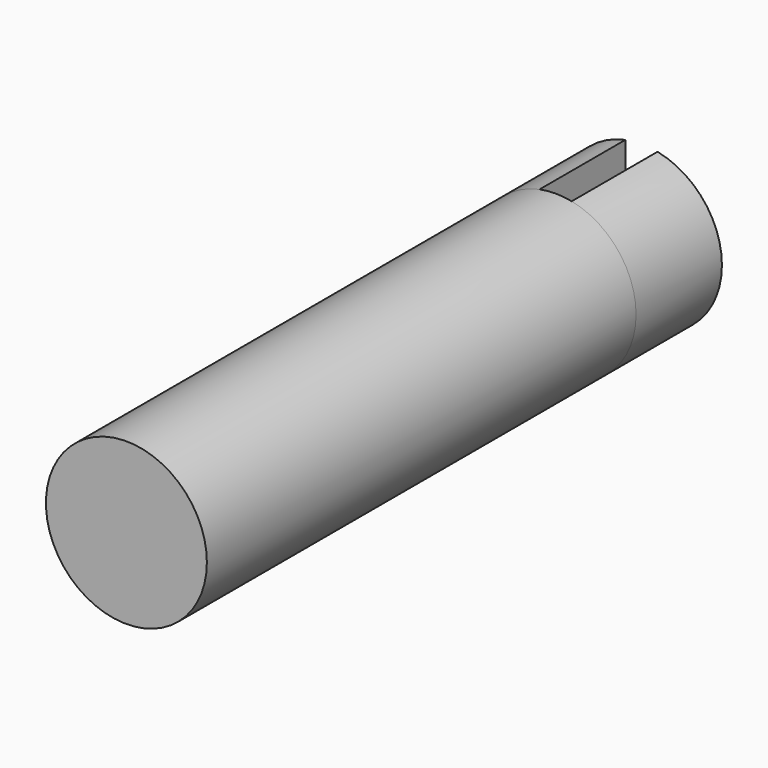
from build123d import *

# Parameters (mm, degrees)
F0_R     = 19.05
F1_DEPTH = 127
F3_DEPTH = 25.4


# Not quite as in the source:
# - after a boolean that leaves OpenCascade's solid faulty, fix() repairs it


with BuildPart() as f1:
    # F0 (on Front) → F1 (new body)
    with BuildSketch(Plane.XZ):
        Circle(F0_R)
    extrude(amount=F1_DEPTH)

    # F2 (on face) → F3 (join)
    with BuildSketch(Plane(origin=(0, 0, 0), x_dir=(-1, 0, 0), z_dir=(0, 1, 0))):
        with BuildLine():
            Line((-3.81, 11.045112), (-3.81, 18.665112))
            ThreePointArc((-3.81, 18.665112), (-19.05, 0), (-3.81, -18.665112))
            Line((-3.81, -18.665112), (-3.81, -11.045112))
            Line((-3.81, -11.045112), (3.81, -11.045112))
            Line((3.81, -11.045112), (3.81, -18.665112))
            ThreePointArc((3.81, -18.665112), (14.756067, -12.048278), (19.05, 0))
            ThreePointArc((19.05, 0), (14.756067, 12.048278), (3.81, 18.665112))
            Line((3.81, 18.665112), (3.81, 11.045112))
            Line((3.81, 11.045112), (-3.81, 11.045112))
        make_face()
    extrude(amount=F3_DEPTH)

    add(f1.part.fix(), mode=Mode.REPLACE)


solid = f1.part
